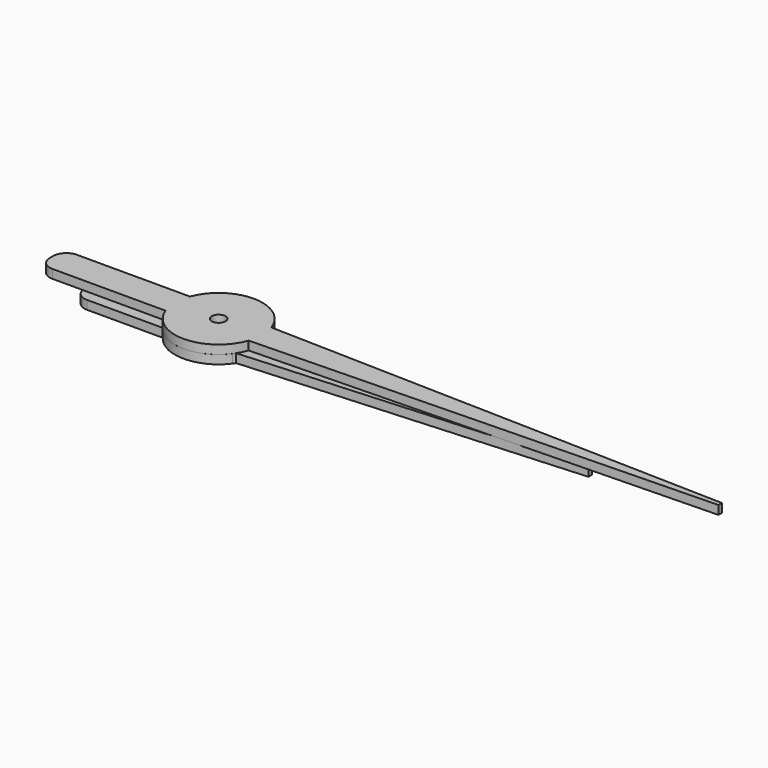
from build123d import *

# Parameters (mm, degrees)
F4_R         = 1.5875
F5_DEPTH     = 2
F6_R         = 1.5875
F7_DEPTH     = 2
F8_T4_DEPTH  = 443.9658863068
F8_S5_R      = 10
F8_T6_DEPTH  = 228
F8_T10_DEPTH = 443.9658863068
F8_S11_R     = 10
F8_T12_DEPTH = 228
F9_T4_DEPTH  = 598.692462338
F9_S5_R      = 10
F9_T6_DEPTH  = 306
F9_T10_DEPTH = 598.692462338
F9_S11_R     = 10
F9_T12_DEPTH = 306
F10_R        = 3
F10_2_R      = 3


# Not quite as in the source:
# - a fillet or chamfer that OpenCascade refuses, or shapes differently, is made with other operations: its cross-section is extruded or revolved along the edge and cut away or added


with BuildPart() as f5:
    # F4 (on Top) → F5 (new body)
    with BuildSketch(Plane.XY):
        with BuildLine():
            Line((-9.3674969976, 3.5), (-38.25, 3.5))
            Line((-38.25, 3.5), (-38.25, -3.5))
            Line((-38.25, -3.5), (-9.3674969976, -3.5))
            ThreePointArc((-9.3674969976, -3.5), (-10, 0), (-9.3674969976, 3.5))
        make_face()
        with BuildLine():
            ThreePointArc((9.3674969976, 3.5), (0, 10), (-9.3674969976, 3.5))
            Line((-9.3674969976, 3.5), (9.3674969976, 3.5))
        make_face()
        with BuildLine():
            Line((9.3674969976, 3.5), (-9.3674969976, 3.5))
            ThreePointArc((-9.3674969976, 3.5), (-10, 0), (-9.3674969976, -3.5))
            Line((-9.3674969976, -3.5), (9.3674969976, -3.5))
            ThreePointArc((9.3674969976, -3.5), (9.8406038935, -1.7783461452), (10, 0))
            ThreePointArc((10, 0), (9.8406038935, 1.7783461452), (9.3674969976, 3.5))
        make_face()
        Circle(F4_R, mode=Mode.SUBTRACT)
        with BuildLine():
            Line((114.75, 3.5), (9.3674969976, 3.5))
            ThreePointArc((9.3674969976, 3.5), (9.8406038935, 1.7783461452), (10, 0))
            ThreePointArc((10, 0), (9.8406038935, -1.7783461452), (9.3674969976, -3.5))
            Line((9.3674969976, -3.5), (114.75, -3.5))
            Line((114.75, -3.5), (114.75, 3.5))
        make_face()
        with BuildLine():
            Line((9.3674969976, -3.5), (-9.3674969976, -3.5))
            ThreePointArc((-9.3674969976, -3.5), (0, -10), (9.3674969976, -3.5))
        make_face()
    extrude(amount=F5_DEPTH)

    # F9: chamfer of 114.75 x 3 on 2 edges, made by hand


with BuildPart() as f7:
    # F6 (on Top) → F7 (new body)
    with BuildSketch(Plane.XY):
        with BuildLine():
            Line((-8, 6), (-28.3333333333, 6))
            Line((-28.3333333333, 6), (-28.3333333333, -6))
            Line((-28.3333333333, -6), (-8, -6))
            ThreePointArc((-8, -6), (-10, 0), (-8, 6))
        make_face()
        with BuildLine():
            ThreePointArc((8, 6), (0, 10), (-8, 6))
            Line((-8, 6), (8, 6))
        make_face()
        with BuildLine():
            Line((8, 6), (-8, 6))
            ThreePointArc((-8, 6), (-10, 0), (-8, -6))
            Line((-8, -6), (8, -6))
            ThreePointArc((8, -6), (9.4868329805, -3.1622776602), (10, 0))
            ThreePointArc((10, 0), (9.4868329805, 3.1622776602), (8, 6))
        make_face()
        Circle(F6_R, mode=Mode.SUBTRACT)
        with BuildLine():
            Line((85, 6), (8, 6))
            ThreePointArc((8, 6), (9.4868329805, 3.1622776602), (10, 0))
            ThreePointArc((10, 0), (9.4868329805, -3.1622776602), (8, -6))
            Line((8, -6), (85, -6))
            Line((85, -6), (85, 6))
        make_face()
        with BuildLine():
            Line((8, -6), (-8, -6))
            ThreePointArc((-8, -6), (0, -10), (8, -6))
        make_face()
    extrude(amount=-F7_DEPTH)

    # F8: chamfer of 85 x 5.5 on 2 edges, made by hand


with BuildPart() as f8_tool2:
    # F8_s3 → F8_t4 (new body)
    with BuildSketch(Plane.XY.offset(220.9829431534)):
        Polygon((0, -6), (85, -0.5), (85, -6), align=None)
    extrude(amount=-F8_T4_DEPTH)

    # F8_s5 → F8_t6 (cut, symmetric)
    with BuildSketch(Plane.XY.offset(-1)):
        Circle(F8_S5_R)
    extrude(amount=F8_T6_DEPTH, both=True, mode=Mode.SUBTRACT)


with BuildPart() as f7_1:
    add(f7.part)

    # F8_t1: cut F8_tool2
    add(f8_tool2.part, mode=Mode.SUBTRACT)


with BuildPart() as f8_tool8:
    # F8_s9 → F8_t10 (new body)
    with BuildSketch(Plane.XY.offset(220.9829431534)):
        Polygon((85, 0.5), (0, 6), (85, 6), align=None)
    extrude(amount=-F8_T10_DEPTH)

    # F8_s11 → F8_t12 (cut, symmetric)
    with BuildSketch(Plane.XY.offset(-1)):
        Circle(F8_S11_R)
    extrude(amount=F8_T12_DEPTH, both=True, mode=Mode.SUBTRACT)


with BuildPart() as f7_2:
    add(f7_1.part)

    # F8_t7: cut F8_tool8
    add(f8_tool8.part, mode=Mode.SUBTRACT)

    # F10#2
    f10_2_edges = [f7_2.edges().sort_by_distance(p)[0] for p in [
        (-28.333333, 6, -1),
        (-28.333333, -6, -1),
    ]]
    fillet(f10_2_edges, radius=F10_2_R)


with BuildPart() as f9_tool2:
    # F9_s3 → F9_t4 (new body)
    with BuildSketch(Plane.XY.offset(-298.346231169)):
        Polygon((0, -3.5), (114.75, -0.5), (114.75, -3.5), align=None)
    extrude(amount=F9_T4_DEPTH)

    # F9_s5 → F9_t6 (cut, symmetric)
    with BuildSketch(Plane.XY.offset(1)):
        Circle(F9_S5_R)
    extrude(amount=F9_T6_DEPTH, both=True, mode=Mode.SUBTRACT)


with BuildPart() as f5_1:
    add(f5.part)

    # F9_t1: cut F9_tool2
    add(f9_tool2.part, mode=Mode.SUBTRACT)


with BuildPart() as f9_tool8:
    # F9_s9 → F9_t10 (new body)
    with BuildSketch(Plane.XY.offset(-298.346231169)):
        Polygon((114.75, 0.5), (0, 3.5), (114.75, 3.5), align=None)
    extrude(amount=F9_T10_DEPTH)

    # F9_s11 → F9_t12 (cut, symmetric)
    with BuildSketch(Plane.XY.offset(1)):
        Circle(F9_S11_R)
    extrude(amount=F9_T12_DEPTH, both=True, mode=Mode.SUBTRACT)


with BuildPart() as f5_2:
    add(f5_1.part)

    # F9_t7: cut F9_tool8
    add(f9_tool8.part, mode=Mode.SUBTRACT)

    # F10
    f10_edges = [f5_2.edges().sort_by_distance(p)[0] for p in [
        (-38.25, 3.5, 1),
        (-38.25, -3.5, 1),
    ]]
    fillet(f10_edges, radius=F10_R)


solid = Compound([f7_2.part, f5_2.part])
